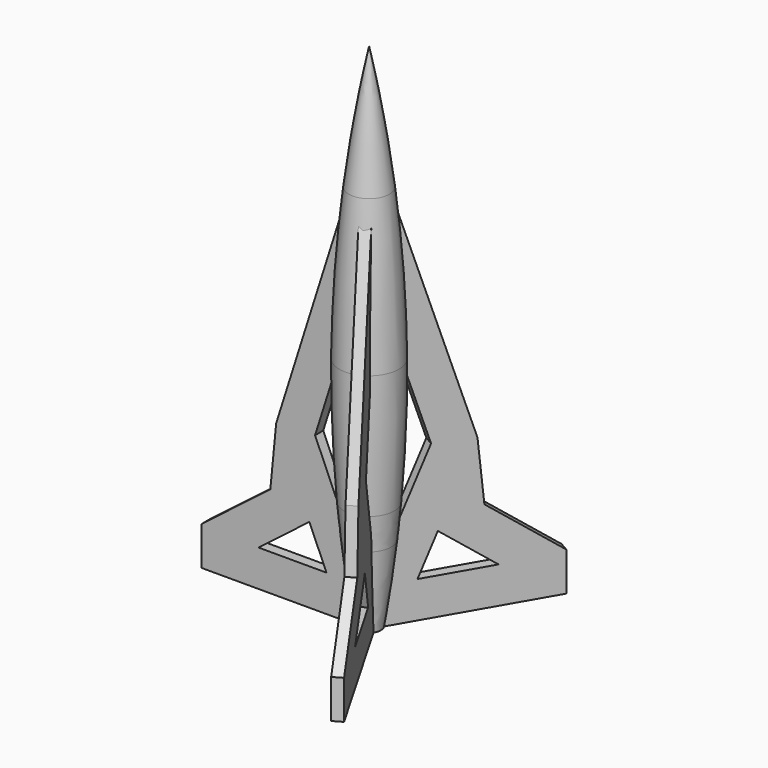
from build123d import *

# Parameters (mm, degrees)
F2_DEPTH      = 0.889
F2_DEPTH_BACK = 0.889
F7_COUNT      = 3


# Not quite as in the source:
# - a feature of the source that left no trace in its solid (it failed there, or was rolled back) is left out
# - a feature names something its author has since deleted; it is built from what else it names


with BuildPart() as f1:
    # F0 (on Front) → F1 (revolve)
    with BuildSketch(Plane.XZ):
        with BuildLine():
            Line((0, 25.4), (0, 19.05))
            Line((0, 19.05), (4.3750425821, 19.05))
            ThreePointArc((4.3750425821, 19.05), (5.0301562728, 30.0344697163), (5.1862594421, 41.0373502799))
            ThreePointArc((5.1862594421, 41.0373502799), (4.7160685687, 54.2084531096), (3.5309804598, 67.3345566967))
            ThreePointArc((3.5309804598, 67.3345566967), (2.0085410115, 78.1570738466), (0, 88.9))
            Line((0, 88.9), (0, 63.5))
            Line((0, 63.5), (0, 25.4))
        make_face()
        with BuildLine():
            Line((0, 19.05), (0, 0))
            Line((0, 0), (2.0423503593, 0))
            ThreePointArc((2.0423503593, 0), (3.0315532972, 6.6552774473), (3.8357292137, 13.3354377333))
            ThreePointArc((3.8357292137, 13.3354377333), (4.1222950388, 16.1911230619), (4.3750425821, 19.05))
            Line((4.3750425821, 19.05), (0, 19.05))
        make_face()
    revolve(axis=Axis((0, 0, 9.525), (0, 0, 1)))


with BuildPart() as f2:
    # F0 (on Front) → F2 (new body, two sides)
    with BuildSketch(Plane.XZ) as f2_sk:
        with BuildLine():
            ThreePointArc((-5.1862594421, 41.0373502799), (-4.7160685687, 54.2084531096), (-3.5309804598, 67.3345566967))
            Line((-3.5309804598, 67.3345566967), (-16.4741296321, 26.4010541141))
            Line((-16.4741296321, 26.4010541141), (-17.487184138, 15.9486530713))
            Line((-17.487184138, 15.9486530713), (-29.4513311237, 6.75473921))
            Line((-29.4513311237, 6.75473921), (-29.4513311237, 0))
            Line((-29.4513311237, 0), (-2.0423503593, 0))
            ThreePointArc((-2.0423503593, 0), (-2.537342767, 3.171862529), (-2.990301487, 6.35))
            Line((-2.990301487, 6.35), (-7.713265307, 6.35))
            Line((-7.713265307, 6.35), (-19.5566457432, 6.35))
            Line((-19.5566457432, 6.35), (-10.6902445927, 13.163434216))
            Line((-10.6902445927, 13.163434216), (-9.700978126, 26.759275721))
            Line((-9.700978126, 26.759275721), (-5.1862594421, 41.0373502799))
        make_face()
        with BuildLine():
            ThreePointArc((-2.990301487, 6.35), (-3.4383539502, 9.8396522078), (-3.8357292137, 13.3354377333))
            Line((-3.8357292137, 13.3354377333), (-9.700978126, 26.759275721))
            Line((-9.700978126, 26.759275721), (-10.6902445927, 13.163434216))
            Line((-10.6902445927, 13.163434216), (-7.713265307, 6.35))
            Line((-7.713265307, 6.35), (-2.990301487, 6.35))
        make_face()
    extrude(amount=F2_DEPTH)
    extrude(f2_sk.sketch, amount=-F2_DEPTH_BACK)


with BuildPart() as f2_1:
    # F6: moved
    add(f2.part.moved(Location((1, 0, 0))))


with BuildPart() as f7_1:
    # F7: instance of F2
    add(f2_1.part.rotate(Axis((0, 0, 9.525), (0, 0, 1)), 1 * 360 / F7_COUNT))


with BuildPart() as f7_2:
    # F7: instance of F2
    add(f2_1.part.rotate(Axis((0, 0, 9.525), (0, 0, 1)), 2 * 360 / F7_COUNT))


solid = Compound([f1.part, f2_1.part, f7_1.part, f7_2.part])
